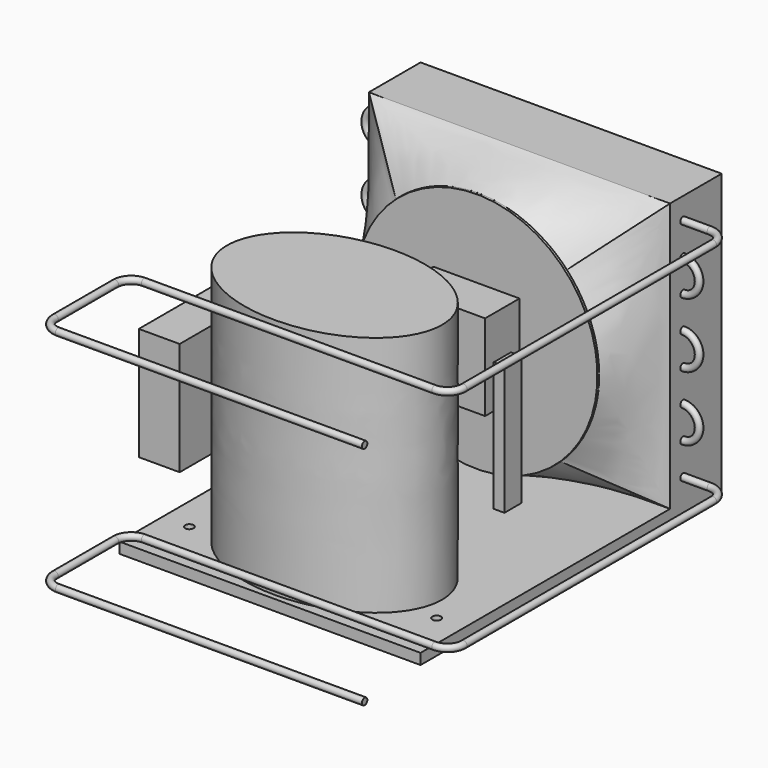
from build123d import *

# Parameters (mm, degrees)
F0_R      = 4
F1_DEPTH  = 10
F0_W      = 280
F0_H      = 60
F2_DEPTH  = 260
F3_DEPTH  = 235
F4_START  = 75
F4_DEPTH  = 105
F0_W_2    = 10
F0_H_2    = 20
F5_DEPTH  = 130
F6_START  = 90
F6_DEPTH  = 80
F7_R      = 112.5
F7_W      = 80
F7_H      = 80
F8_DEPTH  = 2
F2_FACE_W = 280
F2_FACE_H = 250
F10_R     = 3.15
F13_W     = 4
F13_H     = 250
F14_DEPTH = 55


# Not quite as in the source:
# - the arcs of a loft's sections are written as splines that run evenly, so that the points pair up as in the source's solid


with BuildPart() as f1:
    # F0 (on Top) → F1 (new body)
    with BuildSketch(Plane.XY):
        Polygon((280, -60), (0, -60), (0, -350), (280, -350), (280, -300), (280, -200), align=None)
        with BuildLine():
            add(Edge.make_bspline(
                [(240, -275), (240, -214.2893218813), (154.1421356237, -205.7035354437), (68.2842712475, -197.1177490061), (44, -255.4)],
                knots=[0, 0, 0, 1.4288992722, 1.4288992722, 2.8577985444, 2.8577985444, 2.8577985444], degree=2, weights=[1, 0.755453955, 1, 0.755453955, 1]))
            add(Edge.make_bspline(
                [(44, -294.6), (68.2842712475, -352.8822509939), (154.1421356237, -344.2964645563), (240, -335.7106781187), (240, -275)],
                knots=[3.4253867628, 3.4253867628, 3.4253867628, 4.854286035, 4.854286035, 6.2831853072, 6.2831853072, 6.2831853072], degree=2, weights=[1, 0.755453955, 1, 0.755453955, 1]))
            Line((44, -294.6), (44, -335))
            Line((44, -335), (6, -335))
            Line((6, -335), (6, -215))
            Line((6, -215), (44, -215))
            Line((44, -215), (44, -255.4))
        make_face(mode=Mode.SUBTRACT)
        with Locations((255, -300)):
            Circle(F0_R, mode=Mode.SUBTRACT)
        Polygon((100, -120), (100, -110), (180, -110), (180, -120), (190, -120), (190, -140), (180, -140), (180, -150), (100, -150), (100, -140), (90, -140), (90, -120), align=None, mode=Mode.SUBTRACT)
        with BuildLine():
            add(Edge.make_bspline(
                [(44, -255.4), (35.8333333333, -275), (44, -294.6)],
                knots=[2.8577985444, 2.8577985444, 2.8577985444, 3.4253867628, 3.4253867628, 3.4253867628], degree=2, weights=[1, 0.96, 1]))
            Line((44, -255.4), (44, -215))
            Line((44, -215), (6, -215))
            Line((6, -215), (6, -335))
            Line((6, -335), (44, -335))
            Line((44, -335), (44, -294.6))
        make_face()
        with Locations((25, -300)):
            Circle(F0_R, mode=Mode.SUBTRACT)
        Polygon((180, -110), (100, -110), (100, -120), (100, -140), (100, -150), (180, -150), (180, -140), (180, -120), align=None)
    extrude(amount=F1_DEPTH)

    # F0 (on Top) → F2 (join)
    with BuildSketch(Plane.XY):
        with Locations((140, -30)):
            Rectangle(F0_W, F0_H)
    extrude(amount=F2_DEPTH)

    # F0 (on Top) → F3 (join)
    with BuildSketch(Plane.XY):
        with BuildLine():
            Line((44, -294.6), (44, -255.4))
            add(Edge.make_bspline(
                [(44, -255.4), (35.8333333333, -275), (44, -294.6)],
                knots=[2.8577985444, 2.8577985444, 2.8577985444, 3.4253867628, 3.4253867628, 3.4253867628], degree=2, weights=[1, 0.96, 1]))
        make_face()
        with BuildLine():
            add(Edge.make_bspline(
                [(44, -294.6), (68.2842712475, -352.8822509939), (154.1421356237, -344.2964645563), (240, -335.7106781187), (240, -275)],
                knots=[3.4253867628, 3.4253867628, 3.4253867628, 4.854286035, 4.854286035, 6.2831853072, 6.2831853072, 6.2831853072], degree=2, weights=[1, 0.755453955, 1, 0.755453955, 1]))
            add(Edge.make_bspline(
                [(240, -275), (240, -214.2893218813), (154.1421356237, -205.7035354437), (68.2842712475, -197.1177490061), (44, -255.4)],
                knots=[0, 0, 0, 1.4288992722, 1.4288992722, 2.8577985444, 2.8577985444, 2.8577985444], degree=2, weights=[1, 0.755453955, 1, 0.755453955, 1]))
            Line((44, -255.4), (44, -294.6))
        make_face()
    extrude(amount=F3_DEPTH)

    # F0 (on Top) → F4 (join)
    with BuildSketch(Plane.XY.offset(F4_START)):
        with BuildLine():
            add(Edge.make_bspline(
                [(44, -255.4), (35.8333333333, -275), (44, -294.6)],
                knots=[2.8577985444, 2.8577985444, 2.8577985444, 3.4253867628, 3.4253867628, 3.4253867628], degree=2, weights=[1, 0.96, 1]))
            Line((44, -255.4), (44, -215))
            Line((44, -215), (6, -215))
            Line((6, -215), (6, -335))
            Line((6, -335), (44, -335))
            Line((44, -335), (44, -294.6))
        make_face()
        with Locations((25, -300)):
            Circle(F0_R, mode=Mode.SUBTRACT)
        with Locations((25, -300)):
            Circle(F0_R)
    extrude(amount=F4_DEPTH)

    # F0 (on Top) → F5 (join)
    with BuildSketch(Plane.XY):
        with Locations((95, -130)):
            Rectangle(F0_W_2, F0_H_2)
        with Locations((185, -130)):
            Rectangle(F0_W_2, F0_H_2)
    extrude(amount=F5_DEPTH)

    # F0 (on Top) → F6 (join)
    with BuildSketch(Plane.XY.offset(F6_START)):
        Polygon((180, -110), (100, -110), (100, -120), (100, -140), (100, -150), (180, -150), (180, -140), (180, -120), align=None)
    extrude(amount=F6_DEPTH)

    # F7 (on face) → F8 (join)
    with BuildSketch(Plane(origin=(0, -110, 0), x_dir=(-1, 0, 0), z_dir=(0, 1, 0))):
        with Locations((-140, 130)):
            Circle(F7_R)
        with Locations((-140, 130)):
            Rectangle(F7_W, F7_H, mode=Mode.SUBTRACT)
        with Locations((-140, 130)):
            Rectangle(F7_W, F7_H)
    extrude(amount=F8_DEPTH)

    # F8_face (on face) → F9 section 0
    with BuildSketch(Plane(origin=(140, -108, 130), x_dir=(-1, 0, 0), z_dir=(0, 1, 0))):
        with BuildLine():
            add(Edge.make_bspline(
                [(-82.439267808, 76.5507486788), (-87.4495025929, 71.1551112181), (-91.9282027249, 65.266154322), (-99.6508584823, 52.7273340872), (-102.8946231499, 46.0777807956), (-108.0226877651, 32.2732750771), (-109.9068609113, 25.1186639939), (-112.2432657369, 10.5789722049), (-112.6954396443, 3.1942510217), (-112.1503979532, -11.5218746364), (-111.1531958321, -18.852915226), (-107.7476532709, -33.179942297), (-105.3393970395, -40.1755745143), (-99.2042266989, -53.5629233826), (-95.4774642937, -59.9543090048), (-86.8484373292, -71.887511361), (-81.9463861395, -77.429033023), (-76.5507486788, -82.439267808)],
                knots=[0, 0, 0, 0, 0.125, 0.125, 0.25, 0.25, 0.375, 0.375, 0.5, 0.5, 0.625, 0.625, 0.75, 0.75, 0.875, 0.875, 1, 1, 1, 1], degree=3))
            add(Edge.make_bspline(
                [(-76.5507486788, -82.439267808), (-71.1551112181, -87.4495025929), (-65.266154322, -91.9282027249), (-52.7273340872, -99.6508584823), (-46.0777807956, -102.8946231499), (-32.2732750771, -108.0226877651), (-25.1186639939, -109.9068609113), (-10.5789722049, -112.2432657369), (-3.1942510217, -112.6954396443), (11.5218746364, -112.1503979532), (18.852915226, -111.1531958321), (33.179942297, -107.7476532709), (40.1755745143, -105.3393970395), (53.5629233826, -99.2042266989), (59.9543090048, -95.4774642937), (71.887511361, -86.8484373292), (77.429033023, -81.9463861395), (82.439267808, -76.5507486788)],
                knots=[0, 0, 0, 0, 0.125, 0.125, 0.25, 0.25, 0.375, 0.375, 0.5, 0.5, 0.625, 0.625, 0.75, 0.75, 0.875, 0.875, 1, 1, 1, 1], degree=3))
            add(Edge.make_bspline(
                [(82.439267808, -76.5507486788), (87.4495025929, -71.1551112181), (91.9282027249, -65.266154322), (99.6508584823, -52.7273340872), (102.8946231499, -46.0777807956), (108.0226877651, -32.2732750771), (109.9068609113, -25.1186639939), (112.2432657369, -10.5789722049), (112.6954396443, -3.1942510217), (112.1503979532, 11.5218746364), (111.1531958321, 18.852915226), (107.7476532709, 33.179942297), (105.3393970395, 40.1755745143), (99.2042266989, 53.5629233826), (95.4774642937, 59.9543090048), (86.8484373292, 71.887511361), (81.9463861395, 77.429033023), (76.5507486788, 82.439267808)],
                knots=[0, 0, 0, 0, 0.125, 0.125, 0.25, 0.25, 0.375, 0.375, 0.5, 0.5, 0.625, 0.625, 0.75, 0.75, 0.875, 0.875, 1, 1, 1, 1], degree=3))
            add(Edge.make_bspline(
                [(76.5507486788, 82.439267808), (71.1551112181, 87.4495025929), (65.266154322, 91.9282027249), (52.7273340872, 99.6508584823), (46.0777807956, 102.8946231499), (32.2732750771, 108.0226877651), (25.1186639939, 109.9068609113), (10.5789722049, 112.2432657369), (3.1942510217, 112.6954396443), (-11.5218746364, 112.1503979532), (-18.852915226, 111.1531958321), (-33.179942297, 107.7476532709), (-40.1755745143, 105.3393970395), (-53.5629233826, 99.2042266989), (-59.9543090048, 95.4774642937), (-71.887511361, 86.8484373292), (-77.429033023, 81.9463861395), (-82.439267808, 76.5507486788)],
                knots=[0, 0, 0, 0, 0.125, 0.125, 0.25, 0.25, 0.375, 0.375, 0.5, 0.5, 0.625, 0.625, 0.75, 0.75, 0.875, 0.875, 1, 1, 1, 1], degree=3))
        make_face()
    # F2_face (on face) → F9 section 1
    with BuildSketch(Plane(origin=(140, -60, 135), x_dir=(1, 0, 0), z_dir=(0, -1, 0))):
        Rectangle(F2_FACE_W, F2_FACE_H)
    loft(ruled=True)

    # F12: sweep along a path in F11
    with BuildLine(Plane.XY.offset(260)) as f12_path:
        Line((280, -45), (305, -45))
        ThreePointArc((305, -45), (315.6066017178, -49.3933982822), (320, -60))
        Line((320, -60), (320, -350))
        ThreePointArc((320, -350), (315.6066017178, -360.6066017178), (305, -365))
        Line((305, -365), (35, -365))
        ThreePointArc((35, -365), (24.3933982822, -369.3933982822), (20, -380))
        Line((20, -380), (20, -450))
        ThreePointArc((20, -450), (24.3933982822, -460.6066017178), (35, -465))
        Line((35, -465), (320, -465))
    # F10 (on face) → F12 (sweep)
    with BuildSketch(Plane.YZ.offset(280)):
        with Locations((-45, 240)):
            Circle(F10_R)
        with Locations((-45, 30)):
            Circle(F10_R)
    sweep(path=f12_path.line)

    # F13 (on face) → F14 (cut)
    with BuildSketch(Plane(origin=(0, 0, 0), x_dir=(-1, 0, 0), z_dir=(0, 1, 0))):
        with Locations((-273, 130)):
            Rectangle(F13_W, F13_H)
        with Locations((-268.49152542, 130)):
            Rectangle(F13_W, F13_H)
        with Locations((-263.98305084, 130)):
            Rectangle(F13_W, F13_H)
        with Locations((-259.47457626, 130)):
            Rectangle(F13_W, F13_H)
        with Locations((-254.96610168, 130)):
            Rectangle(F13_W, F13_H)
        with Locations((-250.4576271, 130)):
            Rectangle(F13_W, F13_H)
        with Locations((-245.94915252, 130)):
            Rectangle(F13_W, F13_H)
        with Locations((-241.44067794, 130)):
            Rectangle(F13_W, F13_H)
        with Locations((-236.93220336, 130)):
            Rectangle(F13_W, F13_H)
        with Locations((-232.42372878, 130)):
            Rectangle(F13_W, F13_H)
        with Locations((-227.9152542, 130)):
            Rectangle(F13_W, F13_H)
        with Locations((-223.40677962, 130)):
            Rectangle(F13_W, F13_H)
        with Locations((-209.88135588, 130)):
            Rectangle(F13_W, F13_H)
        with Locations((-196.35593214, 130)):
            Rectangle(F13_W, F13_H)
        with Locations((-182.8305084, 130)):
            Rectangle(F13_W, F13_H)
        with Locations((-169.30508466, 130)):
            Rectangle(F13_W, F13_H)
        with Locations((-160.2881355, 130)):
            Rectangle(F13_W, F13_H)
        with Locations((-151.27118634, 130)):
            Rectangle(F13_W, F13_H)
        with Locations((-142.25423718, 130)):
            Rectangle(F13_W, F13_H)
        with Locations((-128.72881344, 130)):
            Rectangle(F13_W, F13_H)
        with Locations((-106.18644054, 130)):
            Rectangle(F13_W, F13_H)
        with Locations((-92.6610168, 130)):
            Rectangle(F13_W, F13_H)
        with Locations((-88.15254222, 130)):
            Rectangle(F13_W, F13_H)
        with Locations((-74.62711848, 130)):
            Rectangle(F13_W, F13_H)
        with Locations((-61.10169474, 130)):
            Rectangle(F13_W, F13_H)
        with Locations((-47.576271, 130)):
            Rectangle(F13_W, F13_H)
        with Locations((-38.55932184, 130)):
            Rectangle(F13_W, F13_H)
        with Locations((-25.0338981, 130)):
            Rectangle(F13_W, F13_H)
        with Locations((-218.89830504, 130)):
            Rectangle(F13_W, F13_H)
        with Locations((-214.38983046, 130)):
            Rectangle(F13_W, F13_H)
        with Locations((-205.3728813, 130)):
            Rectangle(F13_W, F13_H)
        with Locations((-200.86440672, 130)):
            Rectangle(F13_W, F13_H)
        with Locations((-191.84745756, 130)):
            Rectangle(F13_W, F13_H)
        with Locations((-187.33898298, 130)):
            Rectangle(F13_W, F13_H)
        with Locations((-178.32203382, 130)):
            Rectangle(F13_W, F13_H)
        with Locations((-173.81355924, 130)):
            Rectangle(F13_W, F13_H)
        with Locations((-164.79661008, 130)):
            Rectangle(F13_W, F13_H)
        with Locations((-155.77966092, 130)):
            Rectangle(F13_W, F13_H)
        with Locations((-146.76271176, 130)):
            Rectangle(F13_W, F13_H)
        with Locations((-137.7457626, 130)):
            Rectangle(F13_W, F13_H)
        with Locations((-133.23728802, 130)):
            Rectangle(F13_W, F13_H)
        with Locations((-124.22033886, 130)):
            Rectangle(F13_W, F13_H)
        with Locations((-119.71186428, 130)):
            Rectangle(F13_W, F13_H)
        with Locations((-115.2033897, 130)):
            Rectangle(F13_W, F13_H)
        with Locations((-110.69491512, 130)):
            Rectangle(F13_W, F13_H)
        with Locations((-101.67796596, 130)):
            Rectangle(F13_W, F13_H)
        with Locations((-97.16949138, 130)):
            Rectangle(F13_W, F13_H)
        with Locations((-83.64406764, 130)):
            Rectangle(F13_W, F13_H)
        with Locations((-79.13559306, 130)):
            Rectangle(F13_W, F13_H)
        with Locations((-70.1186439, 130)):
            Rectangle(F13_W, F13_H)
        with Locations((-65.61016932, 130)):
            Rectangle(F13_W, F13_H)
        with Locations((-56.59322016, 130)):
            Rectangle(F13_W, F13_H)
        with Locations((-52.08474558, 130)):
            Rectangle(F13_W, F13_H)
        with Locations((-43.06779642, 130)):
            Rectangle(F13_W, F13_H)
        with Locations((-34.05084726, 130)):
            Rectangle(F13_W, F13_H)
        with Locations((-29.54237268, 130)):
            Rectangle(F13_W, F13_H)
        with Locations((-20.52542352, 130)):
            Rectangle(F13_W, F13_H)
        with Locations((-16.01694894, 130)):
            Rectangle(F13_W, F13_H)
        with Locations((-11.50847436, 130)):
            Rectangle(F13_W, F13_H)
        with Locations((-6.99999978, 130)):
            Rectangle(F13_W, F13_H)
    extrude(amount=-F14_DEPTH, mode=Mode.SUBTRACT)

    # F16: sweep along a path in F15
    with BuildLine(Plane(origin=(0, 0, 0), x_dir=(-1, 0, 0), z_dir=(0, 1, 0))) as f16_path:
        Line((-280, 240), (0, 240))
        ThreePointArc((0, 240), (10.6066017178, 235.6066017178), (15, 225))
        ThreePointArc((15, 225), (10.6066017178, 214.3933982822), (0, 210))
        Line((0, 210), (-280, 210))
        ThreePointArc((-280, 210), (-290.6066017178, 205.6066017178), (-295, 195))
        ThreePointArc((-295, 195), (-290.6066017178, 184.3933982822), (-280, 180))
        Line((-280, 180), (0, 180))
        ThreePointArc((0, 180), (10.6066017178, 175.6066017178), (15, 165))
        ThreePointArc((15, 165), (10.6066017178, 154.3933982822), (0, 150))
        Line((0, 150), (-280, 150))
        ThreePointArc((-280, 150), (-290.6066017178, 145.6066017178), (-295, 135))
        ThreePointArc((-295, 135), (-290.6066017178, 124.3933982822), (-280, 120))
        Line((-280, 120), (0, 120))
        ThreePointArc((0, 120), (10.6066017178, 115.6066017178), (15, 105))
        ThreePointArc((15, 105), (10.6066017178, 94.3933982822), (0, 90))
        Line((0, 90), (-280, 90))
        ThreePointArc((-280, 90), (-290.6066017178, 85.6066017178), (-295, 75))
        ThreePointArc((-295, 75), (-290.6066017178, 64.3933982822), (-280, 60))
        Line((-280, 60), (0, 60))
        ThreePointArc((0, 60), (10.6066017178, 55.6066017178), (15, 45))
        ThreePointArc((15, 45), (10.6066017178, 34.3933982822), (0, 30))
        Line((0, 30), (-280, 30))
    # F10 (on face) → F16 (sweep)
    with BuildSketch(Plane.YZ.offset(280)):
        with Locations((-45, 240)):
            Circle(F10_R)
    sweep(path=f16_path.line)


solid = f1.part
